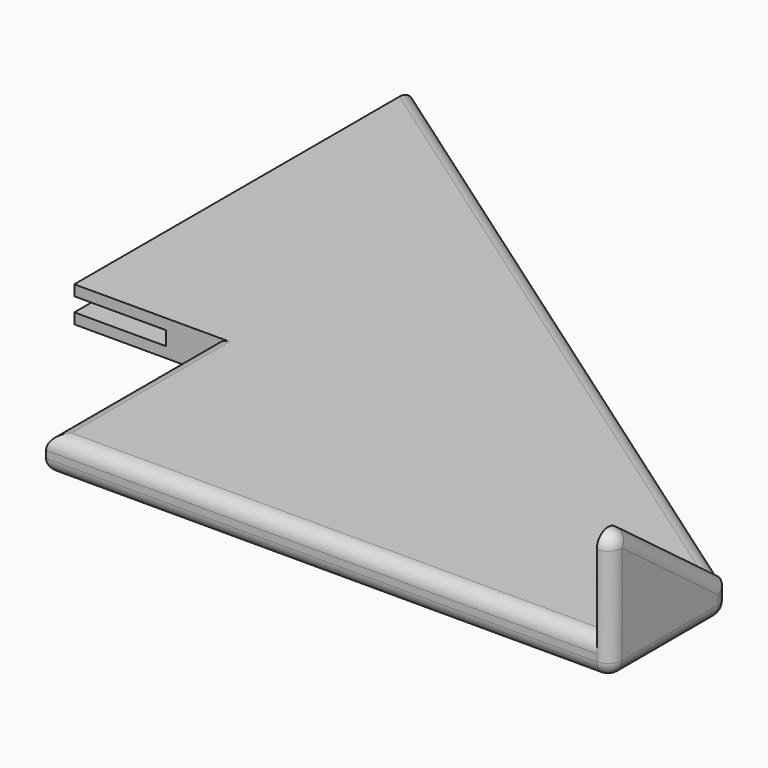
from build123d import *

# Parameters (mm, degrees)
F1_DEPTH     = 12.7
F3_DEPTH     = 5.08
F4_T1_DEPTH  = 335.4465126396
F4_T3_DEPTH  = 88.9
F4_T5_DEPTH  = 210.82
F4_T7_DEPTH  = 228.6
F4_T12_DEPTH = 335.4465126396
F4_T17_DEPTH = 335.4465126396
F5_W         = 33.02
F5_H         = 5.08
F6_DEPTH     = 152.401
F7_T1_DEPTH  = 25.4
F7_T3_DEPTH  = 66.04
F7_T5_DEPTH  = 35.56
F7_T7_DEPTH  = 43.0750697472
F7_T9_DEPTH  = 14.232325632
F7_T14_DEPTH = 5.08
F7_T20_DEPTH = 5.08
F7_T24_ANGLE = 89.9999999979


# Not quite as in the source:
# - a fillet or chamfer that OpenCascade refuses, or shapes differently, is made with other operations: its cross-section is extruded or revolved along the edge and cut away or added


with BuildPart() as f1:
    # F0 (on Top) → F1 (new body)
    with BuildSketch(Plane.XY):
        Polygon((-173.2576622277, 152.4), (-173.2576622277, 0), (-122.4576622277, 0), (-122.4576622277, -76.2), (80.7423377723, -76.2), (80.7423377723, -25.4), align=None)
    extrude(amount=F1_DEPTH)

    # F2 (on face) → F3 (join)
    with BuildSketch(Plane.YZ.offset(80.7423377723)):
        Polygon((-76.2, 12.7), (-25.4, 12.7), (-76.2, 50.8), align=None)
    extrude(amount=-F3_DEPTH)

    # F4: fillet of radius 5.08 on 6 edges, made by hand

    # F4_s2 → F4_t1 (cut)
    with BuildSketch(Plane(origin=(76.5266197344, -53.5686338141, 0), x_dir=(0, 0, 1), z_dir=(-0.8192319205, 0.5734623444, 0))):
        with BuildLine():
            ThreePointArc((5.08, 25.4941995271), (1.4878975516, 24.0063019755), (0, 20.4141995271))
            Line((0, 20.4141995271), (0, 25.4941995271))
            Line((0, 25.4941995271), (5.08, 25.4941995271))
        make_face()
    extrude(amount=F4_T1_DEPTH, mode=Mode.SUBTRACT)

    # F4_s4 → F4_t3 (cut)
    with BuildSketch(Plane.XZ):
        with BuildLine():
            ThreePointArc((-117.3776622277, 12.7), (-120.9697646762, 11.2121024484), (-122.4576622277, 7.62))
            Line((-122.4576622277, 7.62), (-122.4576622277, 12.7))
            Line((-122.4576622277, 12.7), (-117.3776622277, 12.7))
        make_face()
        with BuildLine():
            ThreePointArc((-122.4576622277, 5.08), (-120.9697646762, 1.4878975516), (-117.3776622277, 0))
            Line((-117.3776622277, 0), (-122.4576622277, 0))
            Line((-122.4576622277, 0), (-122.4576622277, 5.08))
        make_face()
    extrude(amount=F4_T3_DEPTH, mode=Mode.SUBTRACT)

    # F4_s6 → F4_t5 (cut)
    with BuildSketch(Plane.YZ.offset(-135.1576622277)):
        with BuildLine():
            ThreePointArc((-71.12, 12.7), (-74.7121024484, 11.2121024484), (-76.2, 7.62))
            Line((-76.2, 7.62), (-76.2, 12.7))
            Line((-76.2, 12.7), (-71.12, 12.7))
        make_face()
    extrude(amount=F4_T5_DEPTH, mode=Mode.SUBTRACT)

    # F4_s8 → F4_t7 (cut)
    with BuildSketch(Plane.YZ.offset(-135.1576622277)):
        with BuildLine():
            ThreePointArc((-76.2, 5.08), (-74.7121024484, 1.4878975516), (-71.12, 0))
            Line((-71.12, 0), (-76.2, 0))
            Line((-76.2, 0), (-76.2, 5.08))
        make_face()
    extrude(amount=F4_T7_DEPTH, mode=Mode.SUBTRACT)


with BuildPart() as f4_tool10:
    # F4_s11 → F4_t12 (new body)
    with BuildSketch(Plane(origin=(76.5266197344, -53.5686338141, 0), x_dir=(0, 0, 1), z_dir=(-0.8192319205, 0.5734623444, 0))):
        with BuildLine():
            ThreePointArc((7.62, 25.4941995271), (11.2121024484, 24.0063019755), (12.7, 20.4141995271))
            Line((12.7, 20.4141995271), (12.7, 25.4941995271))
            Line((12.7, 25.4941995271), (7.62, 25.4941995271))
        make_face()
    extrude(amount=F4_T12_DEPTH)

    split(bisect_by=Plane.YZ.offset(75.6623377723), keep=Keep.BOTTOM)


with BuildPart() as f1_1:
    add(f1.part)

    # F4_t9: cut F4_tool10
    add(f4_tool10.part, mode=Mode.SUBTRACT)


with BuildPart() as f4_tool15:
    # F4_s16 → F4_t17 (new body)
    with BuildSketch(Plane(origin=(76.5266197344, -53.5686338141, 0), x_dir=(0, 0, 1), z_dir=(-0.8192319205, 0.5734623444, 0))):
        with BuildLine():
            ThreePointArc((7.62, 25.4941995271), (11.2121024484, 24.0063019755), (12.7, 20.4141995271))
            Line((12.7, 20.4141995271), (12.7, 25.4941995271))
            Line((12.7, 25.4941995271), (7.62, 25.4941995271))
        make_face()
    extrude(amount=F4_T17_DEPTH)

    split(bisect_by=Plane(origin=(0, -3.048, -4.064), x_dir=(1, 0, 0), z_dir=(0, 0.6, 0.8)), keep=Keep.TOP)


with BuildPart() as f1_2:
    add(f1_1.part)

    # F4_t14: cut F4_tool15
    add(f4_tool15.part, mode=Mode.SUBTRACT)

    # F5 (on face) → F6 (cut, through all)
    with BuildSketch(Plane.XZ):
        with Locations((-156.7476622277, 6.35)):
            Rectangle(F5_W, F5_H)
    extrude(amount=-F6_DEPTH, mode=Mode.SUBTRACT)

    # F7: fillet of radius 5.08 on 5 edges, made by hand

    # F7_s2 → F7_t1 (cut)
    with BuildSketch(Plane.YZ.offset(50.2623377723)):
        with BuildLine():
            ThreePointArc((-68.072, 44.704), (-73.3918450651, 45.1836901303), (-76.2, 40.64))
            Line((-76.2, 40.64), (-76.2, 50.8))
            Line((-76.2, 50.8), (-68.072, 44.704))
        make_face()
    extrude(amount=F7_T1_DEPTH, mode=Mode.SUBTRACT)

    # F7_s4 → F7_t3 (cut)
    with BuildSketch(Plane(origin=(0, -12.192, 9.144), x_dir=(1, 0, 0), z_dir=(0, -0.8, 0.6))):
        with BuildLine():
            ThreePointArc((75.6623377723, -5.08), (79.2544402207, -6.5678975516), (80.7423377723, -10.16))
            Line((80.7423377723, -10.16), (80.7423377723, -5.08))
            Line((80.7423377723, -5.08), (75.6623377723, -5.08))
        make_face()
    extrude(amount=F7_T3_DEPTH, mode=Mode.SUBTRACT)

    # F7_s6 → F7_t5 (cut)
    with BuildSketch(Plane.XY.offset(5.08)):
        with BuildLine():
            ThreePointArc((80.7423377723, -71.12), (79.2544402207, -74.7121024484), (75.6623377723, -76.2))
            Line((75.6623377723, -76.2), (80.7423377723, -76.2))
            Line((80.7423377723, -76.2), (80.7423377723, -71.12))
        make_face()
    extrude(amount=F7_T5_DEPTH, mode=Mode.SUBTRACT)

    # F7_s8 → F7_t7 (cut)
    with BuildSketch(Plane.XZ.offset(28.0449302528)):
        with BuildLine():
            ThreePointArc((80.7423377723, 5.08), (79.2544402207, 1.4878975516), (75.6623377723, 0))
            Line((75.6623377723, 0), (80.7423377723, 0))
            Line((80.7423377723, 0), (80.7423377723, 5.08))
        make_face()
    extrude(amount=F7_T7_DEPTH, mode=Mode.SUBTRACT)

    # F7_s10 → F7_t9 (cut)
    with BuildSketch(Plane.XY.offset(5.08)):
        with BuildLine():
            ThreePointArc((78.5755264816, -23.8832320966), (80.1681894478, -25.6989335183), (80.7423377723, -28.0449302528))
            Line((80.7423377723, -28.0449302528), (80.7423377723, -25.4))
            Line((80.7423377723, -25.4), (78.5755264816, -23.8832320966))
        make_face()
    extrude(amount=F7_T9_DEPTH, mode=Mode.SUBTRACT)


with BuildPart() as f7_tool12:
    # F7_s13 → F7_t14 (new body)
    with BuildSketch(Plane.XY.offset(5.08)):
        Polygon((75.6623377723, -28.0449302528), (78.5755264816, -23.8832320966), (80.7423377723, -25.4), (80.7423377723, -28.0449302528), align=None)
    extrude(amount=-F7_T14_DEPTH)

    # F7_s15 → F7_t16 (revolve, cut)
    with BuildSketch(Plane(origin=(75.6623377723, -28.0449302528, 5.08), x_dir=(-0.8869786763, -0.4618103808, 0), z_dir=(0.4618103808, -0.8869786763, 0))):
        with BuildLine():
            ThreePointArc((0, -5.08), (5.08, 0), (0, 5.08))
            Line((0, 5.08), (0, -5.08))
        make_face()
    revolve(axis=Axis((75.6623377723, -28.0449302528, 5.08), (0, 0, -1)), mode=Mode.SUBTRACT)


with BuildPart() as f1_3:
    add(f1_2.part)

    # F7_t11: cut F7_tool12
    add(f7_tool12.part, mode=Mode.SUBTRACT)


with BuildPart() as f7_tool18:
    # F7_s19 → F7_t20 (new body)
    with BuildSketch(Plane.YZ.offset(75.6623377723)):
        Polygon((-71.12, 40.64), (-68.072, 44.704), (-76.2, 50.8), (-76.2, 40.64), align=None)
    extrude(amount=F7_T20_DEPTH)

    # F7_s21 → F7_t22 (revolve, cut)
    with BuildSketch(Plane(origin=(75.6623377723, -71.12, 40.64), x_dir=(0, 0.4472135955, -0.894427191), z_dir=(0, -0.894427191, -0.4472135955))):
        with BuildLine():
            ThreePointArc((0, -5.08), (5.08, 0), (0, 5.08))
            Line((0, 5.08), (0, -5.08))
        make_face()
    revolve(axis=Axis((75.6623377723, -71.12, 40.64), (1, 0, 0)), mode=Mode.SUBTRACT)


with BuildPart() as f1_4:
    add(f1_3.part)

    # F7_t17: cut F7_tool18
    add(f7_tool18.part, mode=Mode.SUBTRACT)

    # F7_s23 → F7_t24 (revolve, cut)
    with BuildSketch(Plane.XZ.offset(71.1199999999)):
        with BuildLine():
            ThreePointArc((80.7423377723, 5.08), (79.2544402207, 1.4878975516), (75.6623377723, 0))
            Line((75.6623377723, 0), (80.7423377723, 0))
            Line((80.7423377723, 0), (80.7423377723, 5.08))
        make_face()
    revolve(axis=Axis((80.7423377723, -71.1199999999, 5.0800000001), (-1, 0, 0)), revolution_arc=F7_T24_ANGLE, mode=Mode.SUBTRACT)


solid = f1_4.part
